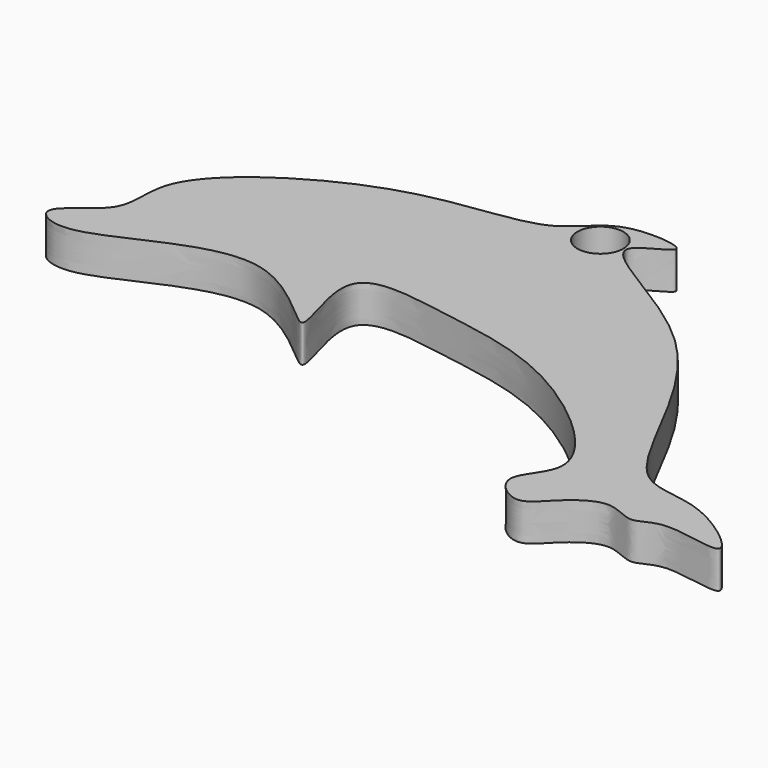
from build123d import *

# Parameters (mm, degrees)
F0_R     = 3.0943943122
F1_DEPTH = 5


# Not quite as in the source:
# - the program builds the solid bodies; features that only make, move or delete a surface that nothing else refers to are left out


with BuildPart() as f1:
    # F0 (on Top) → F1 (new body)
    with BuildSketch(Plane.XY):
        with BuildLine():
            add(Edge.make_bspline(
                [(-38.7898944318, 0), (-36.5886882717, 5.2347176768), (-19.2139289512, 16.3133936998), (-0.8496075829, 15.2846860975), (2.8974058921, 23.3220585712), (15.7022032629, 21.8677639262), (1.5752223201, 17.5670170363), (30.7898114217, 7.4692346629), (39.182588697, -24.1041420173), (49.9735628463, -21.3549558985), (62.5317234873, -31.4198025545), (49.7005662866, -27.2520036037), (46.8728615526, -30.6635989566), (42.559758737, -27.2648560936), (37.5130428154, -31.0999311465), (34.6854600743, -34.9065871525), (28.7752852503, -30.0587139408), (37.6484838484, -23.9909281016), (18.8046505453, -7.6417127836), (3.4591141292, -5.6498348987), (-13.8575631831, -2.3289440703), (-4.431511047, -22.7950835488), (-20.6722083593, -1.8742089512), (-39.6956522123, -17.5582357267), (-47.5529982153, -12.5540963539), (-37.9033616866, -8.3495309393), (-40.0604030422, -3.0214134421), (-38.7898944318, 0)],
                knots=[0, 0, 0, 0, 0.0614112523, 0.1137107326, 0.1484825097, 0.1817604444, 0.2094552348, 0.2678675768, 0.3365840409, 0.3748072417, 0.412615685, 0.4471747281, 0.4718045745, 0.4969940691, 0.5269496065, 0.5520194379, 0.578839213, 0.6100898948, 0.6656032315, 0.719761586, 0.7616164467, 0.801077971, 0.8470414407, 0.9056266474, 0.9318702786, 0.9645541948, 1, 1, 1, 1], degree=3))
        make_face()
        with Locations((4.3930723332, 18.0396381766)):
            Circle(F0_R, mode=Mode.SUBTRACT)
    extrude(amount=F1_DEPTH)


solid = f1.part
